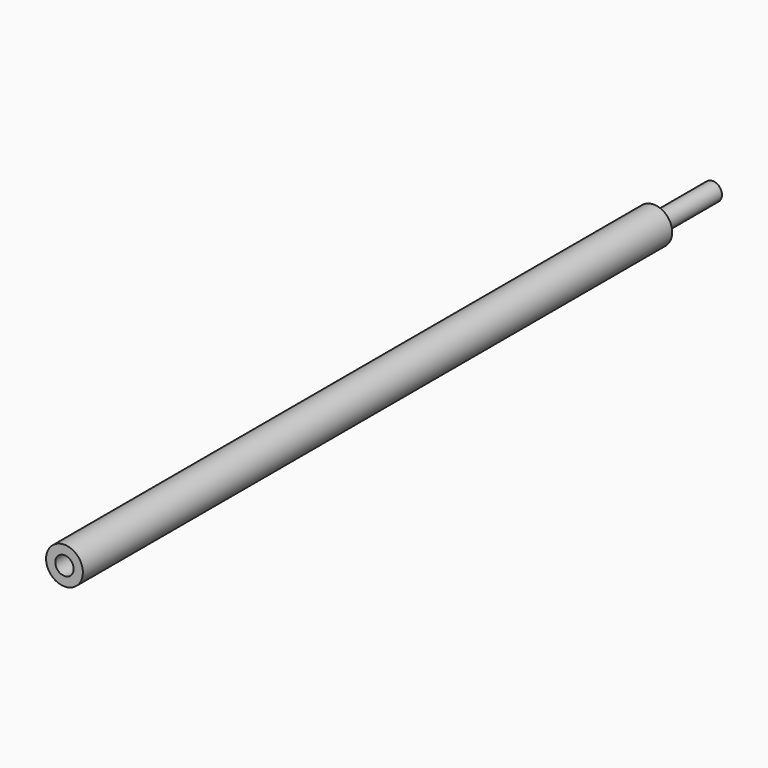
from build123d import *

# Parameters (mm, degrees)
F0_R     = 6.35
F1_DEPTH = 279.4
F2_R     = 6.35
F2_R_2   = 3.175
F3_DEPTH = 25.4
F4_R     = 3.175
F5_DEPTH = 25.4


with BuildPart() as f1:
    # F0 (on Front) → F1 (new body)
    with BuildSketch(Plane.XZ):
        Circle(F0_R)
    extrude(amount=F1_DEPTH)

    # F2 (on face) → F3 (cut)
    with BuildSketch(Plane(origin=(0, 0, 0), x_dir=(-1, 0, 0), z_dir=(0, 1, 0))):
        Circle(F2_R)
        Circle(F2_R_2, mode=Mode.SUBTRACT)
    extrude(amount=-F3_DEPTH, mode=Mode.SUBTRACT)

    # F4 (on face) → F5 (cut)
    with BuildSketch(Plane.XZ.offset(279.4)):
        Circle(F4_R)
    extrude(amount=-F5_DEPTH, mode=Mode.SUBTRACT)


solid = f1.part
